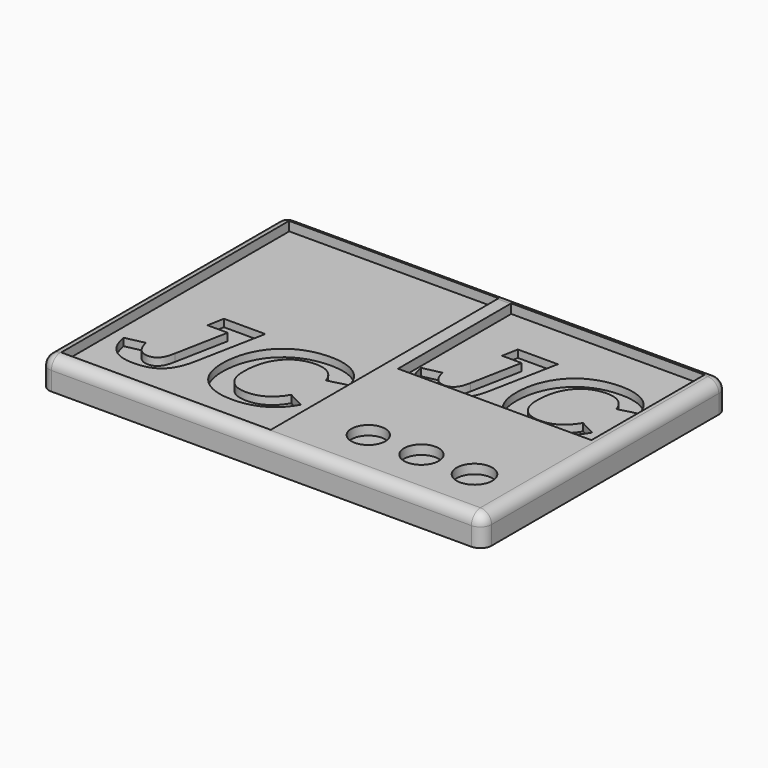
from build123d import *

# Parameters (mm, degrees)
F0_W          = 118.6872683465
F0_H          = 82.2036378086
F1_DEPTH      = 8
F2_W          = 56.2228460331
F2_H          = 76.4822177589
F3_DEPTH      = 2.5
F4_W          = 51.8831089139
F4_H          = 37.9716288298
F5_DEPTH      = 2.5
F6_R          = 4.5524394737
F6_R_2        = 4.6442963165
F6_R_3        = 4.7847285334
F7_DEPTH      = 2.5
F8_T1_DEPTH   = 76.2036378086
F8_T3_DEPTH   = 112.6872683465
F8_T5_DEPTH   = 12.5
F8_S9_W       = 3
F8_S9_H       = 3
F8_T10_DEPTH  = 3
F8_S15_W      = 3
F8_S15_H      = 3
F8_T16_DEPTH  = 3
F8_S21_W      = 3
F8_S21_H      = 3
F8_T22_DEPTH  = 3
F8_S27_W      = 3
F8_S27_H      = 3
F8_T28_DEPTH  = 3
F9_TEXT_SIZE  = 39.4925256158
F10_DEPTH     = 2
F11_TEXT_SIZE = 38.1668847183
F12_DEPTH     = 2


# Not quite as in the source:
# - a fillet or chamfer that OpenCascade refuses, or shapes differently, is made with other operations: its cross-section is extruded or revolved along the edge and cut away or added
# - Text() gives the source's letters only with a copy of the font that has no kerning and outlines rounded to 1/6400 em; it was checked with that copy


with BuildPart() as f1:
    # F0 (on Top) → F1 (new body)
    with BuildSketch(Plane.XY):
        with Locations((-3.4636352211, 11.1990924925)):
            Rectangle(F0_W, F0_H)
    extrude(amount=F1_DEPTH)

    # F2 (on face) → F3 (cut)
    with BuildSketch(Plane.XY.offset(8)):
        with Locations((-31.6045967629, 11.4966686815)):
            Rectangle(F2_W, F2_H)
    extrude(amount=-F3_DEPTH, mode=Mode.SUBTRACT)

    # F4 (on face) → F5 (cut)
    with BuildSketch(Plane.XY.offset(8)):
        with Locations((25.9415544569, 30.5504845455)):
            Rectangle(F4_W, F4_H)
    extrude(amount=-F5_DEPTH, mode=Mode.SUBTRACT)

    # F6 (on face) → F7 (cut)
    with BuildSketch(Plane.XY.offset(8)):
        with Locations((13.9374313876, -15.8028006554)):
            Circle(F6_R)
        with Locations((28.176760301, -15.8028006554)):
            Circle(F6_R_2)
        with Locations((42.4230694771, -15.8028006554)):
            Circle(F6_R_3)
    extrude(amount=-F7_DEPTH, mode=Mode.SUBTRACT)

    # F8: fillet of radius 3 on 8 edges, made by hand

    # F8_s2 → F8_t1 (cut)
    with BuildSketch(Plane.XZ.offset(-49.3009113967)):
        with BuildLine():
            ThreePointArc((55.8799989522, 5), (55.0013192957, 7.1213203436), (52.8799989522, 8))
            Line((52.8799989522, 8), (55.8799989522, 8))
            Line((55.8799989522, 8), (55.8799989522, 5))
        make_face()
        with BuildLine():
            ThreePointArc((-62.8072693944, 5), (-61.928589738, 7.1213203436), (-59.8072693944, 8))
            Line((-59.8072693944, 8), (-62.8072693944, 8))
            Line((-62.8072693944, 8), (-62.8072693944, 5))
        make_face()
    extrude(amount=F8_T1_DEPTH, mode=Mode.SUBTRACT)

    # F8_s4 → F8_t3 (cut)
    with BuildSketch(Plane.YZ.offset(-59.8072693944)):
        with BuildLine():
            ThreePointArc((52.3009113967, 5), (51.4222317403, 7.1213203436), (49.3009113967, 8))
            Line((49.3009113967, 8), (52.3009113967, 8))
            Line((52.3009113967, 8), (52.3009113967, 5))
        make_face()
        with BuildLine():
            ThreePointArc((-26.9027264118, 8), (-29.0240467554, 7.1213203436), (-29.9027264118, 5))
            Line((-29.9027264118, 5), (-29.9027264118, 8))
            Line((-29.9027264118, 8), (-26.9027264118, 8))
        make_face()
    extrude(amount=F8_T3_DEPTH, mode=Mode.SUBTRACT)

    # F8_s6 → F8_t5 (cut)
    with BuildSketch(Plane.XY.offset(-7.5)):
        with BuildLine():
            ThreePointArc((55.8799989522, -26.9027264118), (55.0013192957, -29.0240467554), (52.8799989522, -29.9027264118))
            Line((52.8799989522, -29.9027264118), (55.8799989522, -29.9027264118))
            Line((55.8799989522, -29.9027264118), (55.8799989522, -26.9027264118))
        make_face()
        with BuildLine():
            ThreePointArc((52.8799989522, 52.3009113967), (55.0013192957, 51.4222317403), (55.8799989522, 49.3009113967))
            Line((55.8799989522, 49.3009113967), (55.8799989522, 52.3009113967))
            Line((55.8799989522, 52.3009113967), (52.8799989522, 52.3009113967))
        make_face()
        with BuildLine():
            ThreePointArc((-62.8072693944, -26.9027264118), (-61.928589738, -29.0240467554), (-59.8072693944, -29.9027264118))
            Line((-59.8072693944, -29.9027264118), (-62.8072693944, -29.9027264118))
            Line((-62.8072693944, -29.9027264118), (-62.8072693944, -26.9027264118))
        make_face()
        with BuildLine():
            ThreePointArc((-59.8072693944, 52.3009113967), (-61.928589738, 51.4222317403), (-62.8072693944, 49.3009113967))
            Line((-62.8072693944, 49.3009113967), (-62.8072693944, 52.3009113967))
            Line((-62.8072693944, 52.3009113967), (-59.8072693944, 52.3009113967))
        make_face()
    extrude(amount=F8_T5_DEPTH, mode=Mode.SUBTRACT)


with BuildPart() as f8_tool8:
    # F8_s9 → F8_t10 (new body)
    with BuildSketch(Plane.YZ.offset(52.8799989522)):
        with Locations((-28.4027264118, 6.5)):
            Rectangle(F8_S9_W, F8_S9_H)
    extrude(amount=F8_T10_DEPTH)

    # F8_s11 → F8_t12 (revolve, cut)
    with BuildSketch(Plane(origin=(52.8799989522, -26.9027264118, 5), x_dir=(0, 0.7071067812, -0.7071067812), z_dir=(0, -0.7071067812, -0.7071067812))):
        with BuildLine():
            ThreePointArc((0, -3), (3, 0), (0, 3))
            Line((0, 3), (0, -3))
        make_face()
    revolve(axis=Axis((52.8799989522, -26.9027264118, 5), (1, 0, 0)), mode=Mode.SUBTRACT)


with BuildPart() as f1_1:
    add(f1.part)

    # F8_t7: cut F8_tool8
    add(f8_tool8.part, mode=Mode.SUBTRACT)


with BuildPart() as f8_tool14:
    # F8_s15 → F8_t16 (new body)
    with BuildSketch(Plane.XZ.offset(-49.3009113967)):
        with Locations((54.3799989522, 6.5)):
            Rectangle(F8_S15_W, F8_S15_H)
    extrude(amount=-F8_T16_DEPTH)

    # F8_s17 → F8_t18 (revolve, cut)
    with BuildSketch(Plane(origin=(52.8799989522, 49.3009113967, 5), x_dir=(-0.7071067812, 0, -0.7071067812), z_dir=(0.7071067812, 0, -0.7071067812))):
        with BuildLine():
            ThreePointArc((0, -3), (3, 0), (0, 3))
            Line((0, 3), (0, -3))
        make_face()
    revolve(axis=Axis((52.8799989522, 49.3009113967, 5), (0, 1, 0)), mode=Mode.SUBTRACT)


with BuildPart() as f1_2:
    add(f1_1.part)

    # F8_t13: cut F8_tool14
    add(f8_tool14.part, mode=Mode.SUBTRACT)


with BuildPart() as f8_tool20:
    # F8_s21 → F8_t22 (new body)
    with BuildSketch(Plane.XZ.offset(-49.3009113967)):
        with Locations((-61.3072693944, 6.5)):
            Rectangle(F8_S21_W, F8_S21_H)
    extrude(amount=-F8_T22_DEPTH)

    # F8_s23 → F8_t24 (revolve, cut)
    with BuildSketch(Plane(origin=(-59.8072693944, 49.3009113967, 5), x_dir=(0.7071067812, 0, -0.7071067812), z_dir=(0.7071067812, 0, 0.7071067812))):
        with BuildLine():
            ThreePointArc((0, -3), (3, 0), (0, 3))
            Line((0, 3), (0, -3))
        make_face()
    revolve(axis=Axis((-59.8072693944, 49.3009113967, 5), (0, 1, 0)), mode=Mode.SUBTRACT)


with BuildPart() as f1_3:
    add(f1_2.part)

    # F8_t19: cut F8_tool20
    add(f8_tool20.part, mode=Mode.SUBTRACT)


with BuildPart() as f8_tool26:
    # F8_s27 → F8_t28 (new body)
    with BuildSketch(Plane.YZ.offset(-59.8072693944)):
        with Locations((-28.4027264118, 6.5)):
            Rectangle(F8_S27_W, F8_S27_H)
    extrude(amount=-F8_T28_DEPTH)

    # F8_s29 → F8_t30 (revolve, cut)
    with BuildSketch(Plane(origin=(-59.8072693944, -26.9027264118, 5), x_dir=(0, 0.7071067812, -0.7071067812), z_dir=(0, 0.7071067812, 0.7071067812))):
        with BuildLine():
            ThreePointArc((0, -3), (3, 0), (0, 3))
            Line((0, 3), (0, -3))
        make_face()
    revolve(axis=Axis((-59.8072693944, -26.9027264118, 5), (-1, 0, 0)), mode=Mode.SUBTRACT)


with BuildPart() as f1_4:
    add(f1_3.part)

    # F8_t25: cut F8_tool26
    add(f8_tool26.part, mode=Mode.SUBTRACT)

    # F9 (on face) → F10 (cut)
    with BuildSketch(Plane.XY.offset(5.5)):
        with Locations((-57.1783257553, -16.9379497618)):
            Text('JC', F9_TEXT_SIZE, font='Arimo', font_style=FontStyle.BOLDITALIC, text_align=(TextAlign.LEFT, TextAlign.BOTTOM))
    extrude(amount=-F10_DEPTH, mode=Mode.SUBTRACT)

    # F11 (on face) → F12 (cut)
    with BuildSketch(Plane.XY.offset(5.5)):
        with Locations((0, 11.5646701306)):
            Text('JC', F11_TEXT_SIZE, font='Arimo', font_style=FontStyle.BOLDITALIC, text_align=(TextAlign.LEFT, TextAlign.BOTTOM))
    extrude(amount=-F12_DEPTH, mode=Mode.SUBTRACT)


solid = f1_4.part
